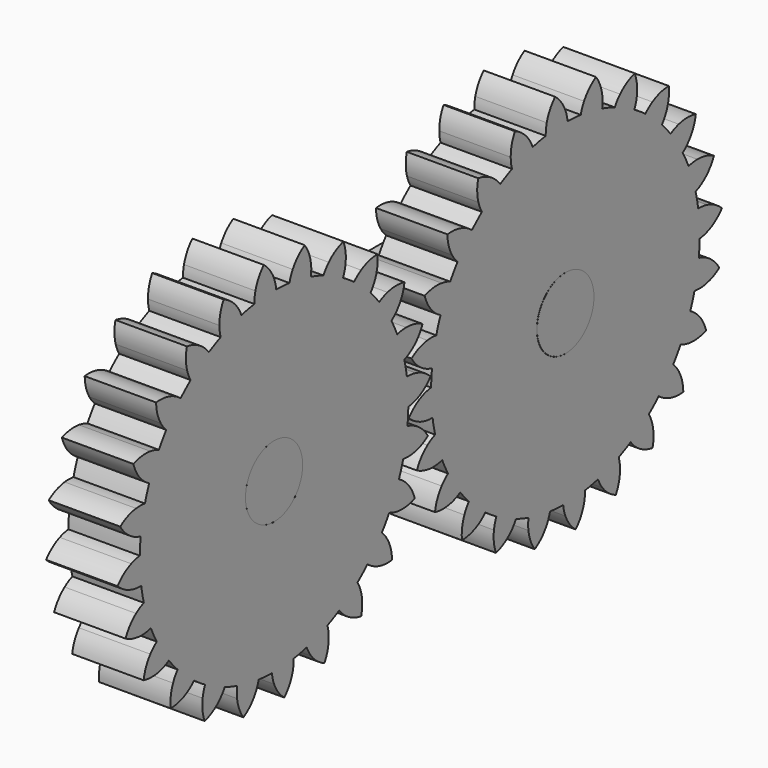
from build123d import *

# Parameters (mm, degrees)
F1_DEPTH = 25.4
F2_DEPTH = 50.8
F3_R     = 22.2127388758
F4_DEPTH = 25.4
F5_COUNT = 24
F3_R_2   = 12.7
F6_DEPTH = 25.4


with BuildPart() as f1:
    # F0 (on Right) → F1 (new body)
    with BuildSketch(Plane.YZ):
        with BuildLine():
            ThreePointArc((12.7, 12.7), (8.9802561211, 3.7197438789), (0, 0))
            Line((0, 0), (129.54, 0))
            ThreePointArc((129.54, 0), (116.84, 12.7), (129.54, 25.4))
            Line((129.54, 25.4), (0, 25.4))
            ThreePointArc((0, 25.4), (8.9802561211, 21.6802561211), (12.7, 12.7))
        make_face()
        with BuildLine():
            ThreePointArc((0, 25.4), (-12.7, 12.7), (0, 0))
            Line((0, 0), (0, 25.4))
        make_face()
        with BuildLine():
            Line((0, 25.4), (0, 0))
            ThreePointArc((0, 0), (8.9802561211, 3.7197438789), (12.7, 12.7))
            ThreePointArc((12.7, 12.7), (8.9802561211, 21.6802561211), (0, 25.4))
        make_face()
        with BuildLine():
            ThreePointArc((129.54, 25.4), (116.84, 12.7), (129.54, 0))
            Line((129.54, 0), (129.54, 25.4))
        make_face()
        with BuildLine():
            Line((129.54, 25.4), (129.54, 0))
            ThreePointArc((129.54, 0), (138.5202561211, 3.7197438789), (142.24, 12.7))
            ThreePointArc((142.24, 12.7), (138.5202561211, 21.6802561211), (129.54, 25.4))
        make_face()
    extrude(amount=F1_DEPTH)

    # F0 (on Right) → F2 (join)
    with BuildSketch(Plane.YZ):
        with BuildLine():
            ThreePointArc((0, 25.4), (-12.7, 12.7), (0, 0))
            Line((0, 0), (0, 25.4))
        make_face()
        with BuildLine():
            Line((0, 25.4), (0, 0))
            ThreePointArc((0, 0), (8.9802561211, 3.7197438789), (12.7, 12.7))
            ThreePointArc((12.7, 12.7), (8.9802561211, 21.6802561211), (0, 25.4))
        make_face()
        with BuildLine():
            ThreePointArc((129.54, 25.4), (116.84, 12.7), (129.54, 0))
            Line((129.54, 0), (129.54, 25.4))
        make_face()
        with BuildLine():
            Line((129.54, 25.4), (129.54, 0))
            ThreePointArc((129.54, 0), (138.5202561211, 3.7197438789), (142.24, 12.7))
            ThreePointArc((142.24, 12.7), (138.5202561211, 21.6802561211), (129.54, 25.4))
        make_face()
    extrude(amount=F2_DEPTH)


with BuildPart() as f4:
    # F3 (on face) → F4 (new body)
    with BuildSketch(Plane.YZ.offset(50.8)):
        with BuildLine():
            ThreePointArc((-8.7423232043, 71.7265883977), (-38.980172643, -32.4786729952), (59.6704814199, 12.7))
            ThreePointArc((59.6704814199, 12.7), (42.5325167196, 54.5515396895), (0.9630155941, 72.3627099104))
            ThreePointArc((0.9630155941, 72.3627099104), (-3.9026362075, 72.2427223388), (-8.7423232043, 71.7265883977))
        make_face()
        with Locations((0, 12.7)):
            Circle(F3_R, mode=Mode.SUBTRACT)
        with BuildLine():
            ThreePointArc((-8.7423232043, 71.7265883977), (-3.9026362075, 72.2427223388), (0.9630155941, 72.3627099104))
            ThreePointArc((0.9630155941, 72.3627099104), (0.6150528404, 74.314869742), (0, 76.2))
            ThreePointArc((0, 76.2), (-1.8836686233, 79.5308162526), (-4.5596046868, 82.2661243844))
            ThreePointArc((-4.5596046868, 82.2661243844), (-6.8556183913, 79.2049374479), (-8.288413206, 75.6567486972))
            ThreePointArc((-8.288413206, 75.6567486972), (-8.6521453097, 73.7074654846), (-8.7423232043, 71.7265883977))
        make_face()
    extrude(amount=F4_DEPTH)


with BuildPart() as f5_1:
    # F5: instance of F4
    add(f4.part.rotate(Axis((50.8, 0, 12.7), (-1, 0, 0)), 1 * 360 / F5_COUNT))


with BuildPart() as f5_2:
    # F5: instance of F4
    add(f4.part.rotate(Axis((50.8, 0, 12.7), (-1, 0, 0)), 2 * 360 / F5_COUNT))


with BuildPart() as f5_3:
    # F5: instance of F4
    add(f4.part.rotate(Axis((50.8, 0, 12.7), (-1, 0, 0)), 3 * 360 / F5_COUNT))


with BuildPart() as f5_4:
    # F5: instance of F4
    add(f4.part.rotate(Axis((50.8, 0, 12.7), (-1, 0, 0)), 4 * 360 / F5_COUNT))


with BuildPart() as f5_5:
    # F5: instance of F4
    add(f4.part.rotate(Axis((50.8, 0, 12.7), (-1, 0, 0)), 5 * 360 / F5_COUNT))


with BuildPart() as f5_6:
    # F5: instance of F4
    add(f4.part.rotate(Axis((50.8, 0, 12.7), (-1, 0, 0)), 6 * 360 / F5_COUNT))


with BuildPart() as f5_7:
    # F5: instance of F4
    add(f4.part.rotate(Axis((50.8, 0, 12.7), (-1, 0, 0)), 7 * 360 / F5_COUNT))


with BuildPart() as f5_8:
    # F5: instance of F4
    add(f4.part.rotate(Axis((50.8, 0, 12.7), (-1, 0, 0)), 8 * 360 / F5_COUNT))


with BuildPart() as f5_9:
    # F5: instance of F4
    add(f4.part.rotate(Axis((50.8, 0, 12.7), (-1, 0, 0)), 9 * 360 / F5_COUNT))


with BuildPart() as f5_10:
    # F5: instance of F4
    add(f4.part.rotate(Axis((50.8, 0, 12.7), (-1, 0, 0)), 10 * 360 / F5_COUNT))


with BuildPart() as f5_11:
    # F5: instance of F4
    add(f4.part.rotate(Axis((50.8, 0, 12.7), (-1, 0, 0)), 11 * 360 / F5_COUNT))


with BuildPart() as f5_12:
    # F5: instance of F4
    add(f4.part.rotate(Axis((50.8, 0, 12.7), (-1, 0, 0)), 12 * 360 / F5_COUNT))


with BuildPart() as f5_13:
    # F5: instance of F4
    add(f4.part.rotate(Axis((50.8, 0, 12.7), (-1, 0, 0)), 13 * 360 / F5_COUNT))


with BuildPart() as f5_14:
    # F5: instance of F4
    add(f4.part.rotate(Axis((50.8, 0, 12.7), (-1, 0, 0)), 14 * 360 / F5_COUNT))


with BuildPart() as f5_15:
    # F5: instance of F4
    add(f4.part.rotate(Axis((50.8, 0, 12.7), (-1, 0, 0)), 15 * 360 / F5_COUNT))


with BuildPart() as f5_16:
    # F5: instance of F4
    add(f4.part.rotate(Axis((50.8, 0, 12.7), (-1, 0, 0)), 16 * 360 / F5_COUNT))


with BuildPart() as f5_17:
    # F5: instance of F4
    add(f4.part.rotate(Axis((50.8, 0, 12.7), (-1, 0, 0)), 17 * 360 / F5_COUNT))


with BuildPart() as f5_18:
    # F5: instance of F4
    add(f4.part.rotate(Axis((50.8, 0, 12.7), (-1, 0, 0)), 18 * 360 / F5_COUNT))


with BuildPart() as f5_19:
    # F5: instance of F4
    add(f4.part.rotate(Axis((50.8, 0, 12.7), (-1, 0, 0)), 19 * 360 / F5_COUNT))


with BuildPart() as f5_20:
    # F5: instance of F4
    add(f4.part.rotate(Axis((50.8, 0, 12.7), (-1, 0, 0)), 20 * 360 / F5_COUNT))


with BuildPart() as f5_21:
    # F5: instance of F4
    add(f4.part.rotate(Axis((50.8, 0, 12.7), (-1, 0, 0)), 21 * 360 / F5_COUNT))


with BuildPart() as f5_22:
    # F5: instance of F4
    add(f4.part.rotate(Axis((50.8, 0, 12.7), (-1, 0, 0)), 22 * 360 / F5_COUNT))


with BuildPart() as f5_23:
    # F5: instance of F4
    add(f4.part.rotate(Axis((50.8, 0, 12.7), (-1, 0, 0)), 23 * 360 / F5_COUNT))


with BuildPart() as f4_1:
    add(f4.part)

    add(f5_1.part)  # F6 merges F5_1

    add(f5_2.part)  # F6 merges F5_2

    add(f5_3.part)  # F6 merges F5_3

    add(f5_4.part)  # F6 merges F5_4

    add(f5_5.part)  # F6 merges F5_5

    add(f5_6.part)  # F6 merges F5_6

    add(f5_7.part)  # F6 merges F5_7

    add(f5_8.part)  # F6 merges F5_8

    add(f5_9.part)  # F6 merges F5_9

    add(f5_10.part)  # F6 merges F5_10

    add(f5_11.part)  # F6 merges F5_11

    add(f5_12.part)  # F6 merges F5_12

    add(f5_13.part)  # F6 merges F5_13

    add(f5_14.part)  # F6 merges F5_14

    add(f5_15.part)  # F6 merges F5_15

    add(f5_16.part)  # F6 merges F5_16

    add(f5_17.part)  # F6 merges F5_17

    add(f5_18.part)  # F6 merges F5_18

    add(f5_19.part)  # F6 merges F5_19

    add(f5_20.part)  # F6 merges F5_20

    add(f5_21.part)  # F6 merges F5_21

    add(f5_22.part)  # F6 merges F5_22

    add(f5_23.part)  # F6 merges F5_23
    # F3 (on face) → F6 (join)
    with BuildSketch(Plane.YZ.offset(50.8)):
        with Locations((0, 12.7)):
            Circle(F3_R)
        with Locations((0, 12.7)):
            Circle(F3_R_2, mode=Mode.SUBTRACT)
    extrude(amount=F6_DEPTH)


with BuildPart() as f7_1:
    # F7: copy of F1
    add(f1.part.moved(Location((25.4, 0, 0))))


with BuildPart() as f9_1:
    # F9: copy of F4
    add(f4_1.part.moved(Location((0, 129.4638, 0))))


solid = Compound([f4_1.part, f7_1.part, f9_1.part])
